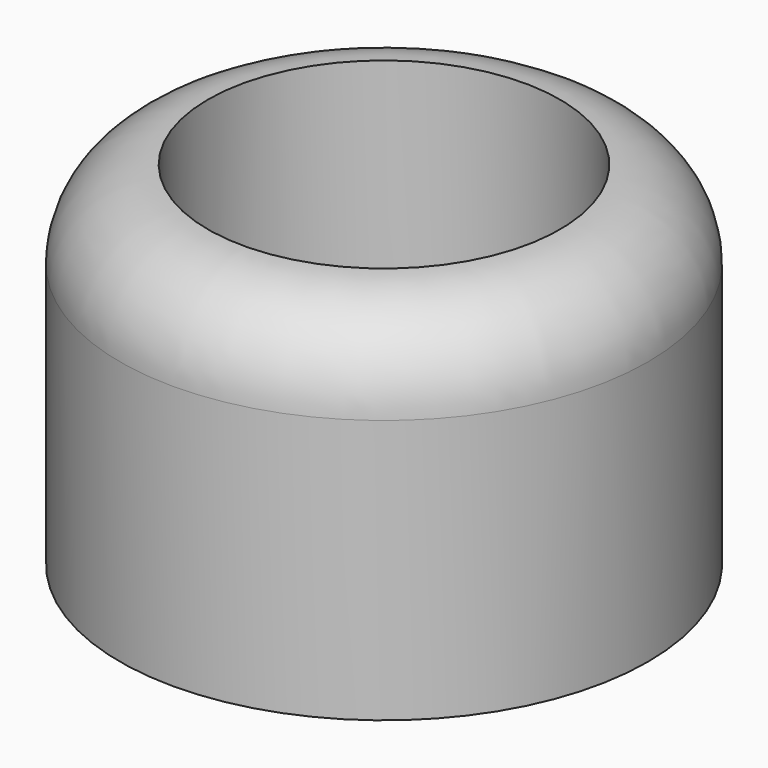
from build123d import *

# Parameters (mm, degrees)
F0_W = 76.2
F0_H = 101.6
F2_R = 25.4
F3_T = -25.4


# Not quite as in the source:
# - a shell that OpenCascade refuses in one call is made with other operations: the cavity is built on its own and cut out


with BuildPart() as f1:
    # F0 (on Front) → F1 (revolve)
    with BuildSketch(Plane.XZ):
        with Locations((-38.1, 0)):
            Rectangle(F0_W, F0_H)
    revolve(axis=Axis((0, 0, 0), (0, 0, -1)))

    # F2
    f2_edges = [f1.edges().sort_by_distance(p)[0] for p in [
        (76.2, 0, 50.8),
    ]]
    fillet(f2_edges, radius=F2_R)

    # F3: a shell. OpenCascade refuses it in one call, so the cavity is built on its own and cut out:
    # the body offset inwards by the wall thickness, plus a prism from it out through each open face.
    f3_core = offset(f1.part, amount=F3_T, kind=Kind.INTERSECTION, mode=Mode.PRIVATE)
    f3_exits = [f3_core.faces().sort_by_distance(p)[0] for p in [
        (0, 0, 25.4),
    ]]
    add(f3_core, mode=Mode.SUBTRACT)
    extrude(f3_exits, amount=-F3_T, mode=Mode.SUBTRACT)


solid = f1.part
